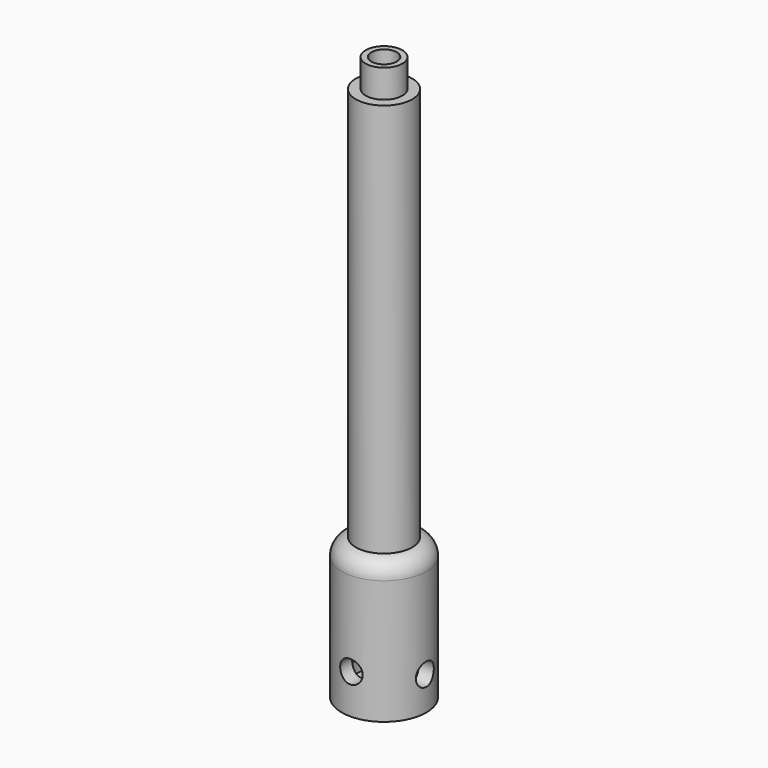
from build123d import *

# Parameters (mm, degrees)
F0_R      = 3.25
F0_R_2    = 2.25
F1_DEPTH  = 80
F0_R_3    = 5
F2_DEPTH  = 75
F0_R_4    = 7.5
F3_DEPTH  = 5
F4_DEPTH  = 20
F6_R      = 5.5
F7_DEPTH  = 2
F8_R      = 2
F9_DEPTH  = 12.5
F10_R     = 2
F11_DEPTH = 12.5


# Not quite as in the source:
# - a fillet or chamfer that OpenCascade refuses, or shapes differently, is made with other operations: its cross-section is extruded or revolved along the edge and cut away or added


with BuildPart() as f1:
    # F0 (on Top) → F1 (new body)
    with BuildSketch(Plane.XY):
        Circle(F0_R)
        Circle(F0_R_2, mode=Mode.SUBTRACT)
    extrude(amount=F1_DEPTH)

    # F0 (on Top) → F2 (join)
    with BuildSketch(Plane.XY):
        Circle(F0_R_3)
        Circle(F0_R, mode=Mode.SUBTRACT)
    extrude(amount=F2_DEPTH)

    # F0 (on Top) → F3 (join)
    with BuildSketch(Plane.XY):
        Circle(F0_R_4)
        Circle(F0_R_3, mode=Mode.SUBTRACT)
    extrude(amount=F3_DEPTH)

    # F0 (on Top) → F4 (join)
    with BuildSketch(Plane.XY):
        Circle(F0_R_4)
        Circle(F0_R_3, mode=Mode.SUBTRACT)
    extrude(amount=-F4_DEPTH)

    # F6 (on offset) → F7 (join)
    with BuildSketch(Plane(origin=(0, 0, -20), x_dir=(1, 0, 0), z_dir=(0, 0, -1))):
        Circle(F6_R)
    extrude(amount=-F7_DEPTH)

    # F8 (on Front) → F9 (cut, symmetric)
    with BuildSketch(Plane.XZ):
        with Locations((0, -13)):
            Circle(F8_R)
    extrude(amount=F9_DEPTH, both=True, mode=Mode.SUBTRACT)

    # F10 (on Right) → F11 (cut, symmetric)
    with BuildSketch(Plane.YZ):
        with Locations((0, -14)):
            Circle(F10_R)
    extrude(amount=F11_DEPTH, both=True, mode=Mode.SUBTRACT)

    # F12: fillet of radius 3 on 1 edges, made by hand

    # F12_s1 → F12_t2 (revolve, cut)
    with BuildSketch(Plane.XZ):
        with BuildLine():
            ThreePointArc((5, 5), (6.7912878475, 3.9784517816), (7.5, 2.0419601084))
            Line((7.5, 2.0419601084), (7.5, 5))
            Line((7.5, 5), (5, 5))
        make_face()
    revolve(axis=Axis((0, 0, 5), (0, 0, 1)), mode=Mode.SUBTRACT)


solid = f1.part
